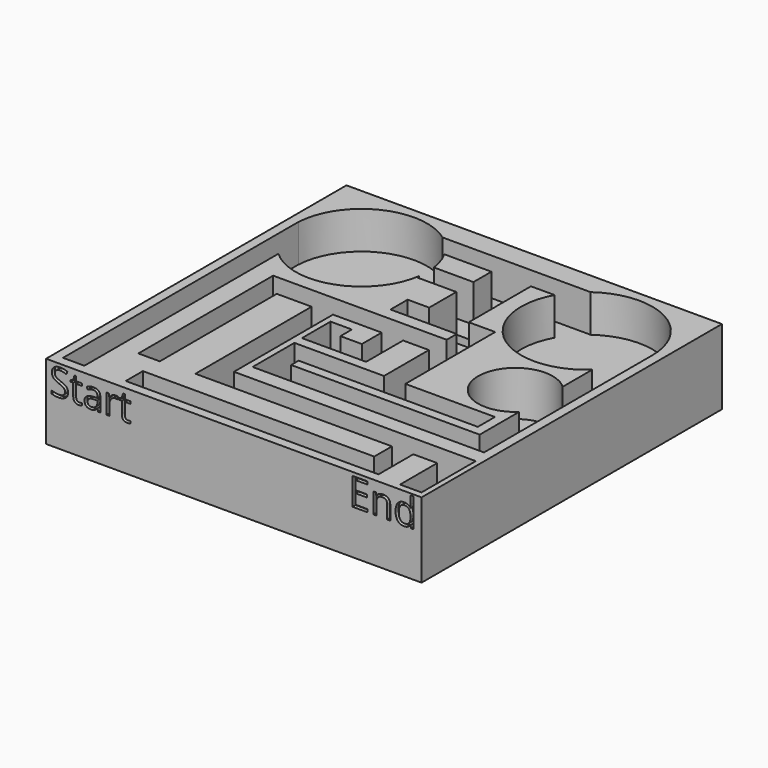
from build123d import *

# Parameters (mm, degrees)
F0_W           = 100
F0_H           = 100
F1_DEPTH       = 20
F2_W           = 10.5249598597
F2_H           = 5.9832503918
F2_W_2         = 17.6280021053
F2_H_2         = 5.7
F2_W_3         = 5.7
F2_H_3         = 38.9400205359
F2_H_4         = 28.7457114801
F2_H_5         = 3.8266098127
F2_H_6         = 12.3720951378
F2_W_4         = 38.370216731
F2_W_5         = 23.2461518608
F3_DEPTH       = 10
F4_R           = 9.9309063048
F4_W           = 10.5430610453
F4_H           = 9.0340993889
F5_DEPTH       = 12
F6_TEXT_SIZE   = 9.8178762772
F6_TEXT_SIZE_2 = 10.1638148971
F7_DEPTH       = 1
F8_TEXT_SIZE   = 18.6877515587
F9_DEPTH       = 1


# Not quite as in the source:
# - Text() gives the source's letters only with a copy of the font that has no kerning and outlines rounded to 1/6400 em; it was checked with that copy


with BuildPart() as f1:
    # F0 (on Top) → F1 (new body)
    with BuildSketch(Plane.XY):
        Rectangle(F0_W, F0_H)
    extrude(amount=-F1_DEPTH)

    # F2 (on face) → F3 (cut)
    with BuildSketch(Plane.XY):
        with BuildLine():
            ThreePointArc((-12.675344194, 27.528906881), (-12.5438910893, 28.7613468212), (-12.5, 30))
            ThreePointArc((-12.5, 30), (-12.5438910893, 31.2386531788), (-12.675344194, 32.471093119))
            Line((-12.675344194, 32.471093119), (-12.675344194, 27.528906881))
        make_face()
        with BuildLine():
            ThreePointArc((-12.675344194, 32.471093119), (-12.5438910893, 31.2386531788), (-12.5, 30))
            ThreePointArc((-12.5, 30), (-12.5438910893, 28.7613468212), (-12.675344194, 27.528906881))
            Line((-12.675344194, 27.528906881), (-12.675344194, 26.771093119))
            Line((-12.675344194, 26.771093119), (2.7480376884, 26.771093119))
            Line((2.7480376884, 26.771093119), (8.3745755255, 26.771093119))
            Line((8.3745755255, 26.771093119), (8.3745755255, 32.471093119))
            Line((8.3745755255, 32.471093119), (-2.1503843342, 32.471093119))
            Line((-2.1503843342, 32.471093119), (-12.675344194, 32.471093119))
        make_face()
        with BuildLine():
            Line((-12.675344194, 27.528906881), (-12.675344194, 32.471093119))
            ThreePointArc((-12.675344194, 32.471093119), (-13.4046274349, 35.553702317), (-14.67766089, 38.4543435108))
            Line((-14.67766089, 38.4543435108), (-19.7090058897, 38.4543435108))
            Line((-19.7090058897, 38.4543435108), (-19.7090058897, 44.1543435108))
            ThreePointArc((-19.7090058897, 44.1543435108), (-37.5622804937, 45.7816955279), (-47.4794772235, 30.8472756296))
            Line((-47.4794772235, 30.8472756296), (-41.8, 30.8472756296))
            Line((-41.8, 30.8472756296), (-41.8, 17.0767651109))
            ThreePointArc((-41.8, 17.0767651109), (-24.0888011081, 13.5285784566), (-12.675344194, 27.528906881))
        make_face()
        with BuildLine():
            Line((-19.7090058897, 38.4543435108), (-14.67766089, 38.4543435108))
            ThreePointArc((-14.67766089, 38.4543435108), (-16.8800453635, 41.5808803783), (-19.7090058897, 44.1543435108))
            Line((-19.7090058897, 44.1543435108), (-19.7090058897, 38.4543435108))
        make_face()
        with BuildLine():
            ThreePointArc((-19.7090058897, 44.1543435108), (-16.8800453635, 41.5808803783), (-14.67766089, 38.4543435108))
            Line((-14.67766089, 38.4543435108), (-2.1503843342, 38.4543435108))
            Line((-2.1503843342, 38.4543435108), (8.3745755255, 38.4543435108))
            Line((8.3745755255, 38.4543435108), (14.67766089, 38.4543435108))
            ThreePointArc((14.67766089, 38.4543435108), (16.8800453635, 41.5808803783), (19.7090058897, 44.1543435108))
            Line((19.7090058897, 44.1543435108), (-19.7090058897, 44.1543435108))
        make_face()
        with Locations((3.1120955956, 35.4627183149)):
            Rectangle(F2_W, F2_H)
        with BuildLine():
            Line((-41.8, 7.7384602059), (-41.8, 17.0767651109))
            ThreePointArc((-41.8, 17.0767651109), (-46.0117144819, 22.9377766002), (-47.5, 30.0000001007))
            Line((-47.5, 30.0000001007), (-47.5, -47.5))
            Line((-47.5, -47.5), (-41.8, -47.5))
            Line((-41.8, -47.5), (-41.8, 2.931000432))
            Line((-41.8, 2.931000432), (-41.8, 7.7384602059))
        make_face()
        with BuildLine():
            ThreePointArc((-47.5, 30.0000001007), (-46.0117144819, 22.9377766002), (-41.8, 17.0767651109))
            Line((-41.8, 17.0767651109), (-41.8, 30.8472756296))
            Line((-41.8, 30.8472756296), (-47.4794772235, 30.8472756296))
            ThreePointArc((-47.4794772235, 30.8472756296), (-47.4948685523, 30.423762123), (-47.5, 30.0000001007))
        make_face()
        with BuildLine():
            Line((-47.5, 30.8472756296), (-47.5, 30.0000001007))
            ThreePointArc((-47.5, 30.0000001007), (-47.4948685523, 30.423762123), (-47.4794772235, 30.8472756296))
            Line((-47.4794772235, 30.8472756296), (-47.5, 30.8472756296))
        make_face()
        with BuildLine():
            Line((19.8722742498, 44.1543435108), (19.7090058897, 44.1543435108))
            ThreePointArc((19.7090058897, 44.1543435108), (16.8800453635, 41.5808803783), (14.67766089, 38.4543435108))
            Line((14.67766089, 38.4543435108), (19.8722742498, 38.4543435108))
            Line((19.8722742498, 38.4543435108), (19.8722742498, 44.1543435108))
        make_face()
        with BuildLine():
            ThreePointArc((47.5, 30), (37.942216412, 45.5939474946), (19.7090058897, 44.1543435108))
            Line((19.7090058897, 44.1543435108), (19.8722742498, 44.1543435108))
            Line((19.8722742498, 44.1543435108), (19.8722742498, 38.4543435108))
            Line((19.8722742498, 38.4543435108), (14.67766089, 38.4543435108))
            ThreePointArc((14.67766089, 38.4543435108), (19.1649092176, 16.2577000565), (41.795897507, 17.0730203835))
            Line((41.795897507, 17.0730203835), (41.795897507, 29.621093119))
            Line((41.795897507, 29.621093119), (47.495897507, 29.621093119))
            ThreePointArc((47.495897507, 29.621093119), (47.4989743467, 29.8105354552), (47.5, 30))
        make_face()
        with BuildLine():
            Line((47.495897507, -0.2311933598), (47.495897507, 29.621093119))
            ThreePointArc((47.495897507, 29.621093119), (45.9331681134, 22.7623101841), (41.795897507, 17.0730203835))
            Line((41.795897507, 17.0730203835), (41.795897507, -0.2311933598))
            Line((41.795897507, -0.2311933598), (47.495897507, -0.2311933598))
        make_face()
        with BuildLine():
            ThreePointArc((41.795897507, 17.0730203835), (45.9331681134, 22.7623101841), (47.495897507, 29.621093119))
            Line((47.495897507, 29.621093119), (41.795897507, 29.621093119))
            Line((41.795897507, 29.621093119), (41.795897507, 17.0730203835))
        make_face()
        Polygon((47.495897507, -26.0778535157), (47.495897507, -0.2311933598), (41.795897507, -0.2311933598), (41.795897507, -20.3778535157), (41.795897507, -26.0778535157), align=None)
        Polygon((41.795897507, -26.0778535157), (41.795897507, -20.3778535157), (-8.432225886, -20.3778535157), (-14.132225886, -20.3778535157), (-14.132225886, -26.0778535157), align=None)
        Polygon((-14.132225886, -20.3778535157), (-8.432225886, -20.3778535157), (-8.432225886, -17.8778535157), (-8.432225886, -12.1778535157), (-14.132225886, -12.1778535157), align=None)
        Polygon((-8.432225886, -12.1778535157), (-8.432225886, -17.8778535157), (39.295897507, -17.8778535157), (39.295897507, -12.1778535157), (32.7667227619, -12.1778535157), (15.4318358105, -12.1778535157), (9.7318358105, -12.1778535157), align=None)
        Polygon((9.7318358105, 2.7795701072), (9.7318358105, -12.1778535157), (15.4318358105, -12.1778535157), (15.4318358105, 17.7369937301), (9.7318358105, 17.7369937301), (9.7318358105, 12.0369937301), (9.7318358105, 8.7082730606), align=None)
        Polygon((2.8549974695, 2.7795701072), (9.7318358105, 2.7795701072), (9.7318358105, 8.7082730606), (-36.4886954397, 8.7082730606), (-36.4886954397, 2.7795701072), (-30.7886954397, 2.7795701072), (-29.9770668119, 2.7795701072), (-26.0700903803, 2.7795701072), (-21.511951831, 2.7795701072), (-15.811951831, 2.7795701072), (-2.8450025305, 2.7795701072), align=None)
        Polygon((2.8549974695, -9.5266098127), (2.8549974695, 2.7795701072), (-2.8450025305, 2.7795701072), (-2.8450025305, -3.8266098127), (-2.8450025305, -9.5266098127), align=None)
        with Locations((0.9178347578, 14.8869937301)):
            Rectangle(F2_W_2, F2_H_2)
        with Locations((-33.6386954397, -16.6904401608)):
            Rectangle(F2_W_3, F2_H_3)
        with Locations((-18.661951831, -11.5932856329)):
            Rectangle(F2_W_3, F2_H_4)
        Polygon((-2.8450025305, -9.5266098127), (-2.8450025305, -3.8266098127), (-8.5450025305, -3.8266098127), (-14.2450025305, -3.8266098127), (-14.2450025305, -9.5266098127), align=None)
        Polygon((-15.811951831, -30.19637205), (-15.811951831, -25.9661413729), (-21.511951831, -25.9661413729), (-21.511951831, -35.89637205), (-15.811951831, -35.89637205), align=None)
        with Locations((-11.3950025305, -1.9133049063)):
            Rectangle(F2_W_3, F2_H_5)
        Polygon((48.5945235908, -30.19637205), (-15.811951831, -30.19637205), (-15.811951831, -35.89637205), (30.8276685918, -35.89637205), (36.5276685918, -35.89637205), (42.8945235908, -35.89637205), (48.5945235908, -35.89637205), align=None)
        Polygon((36.5276685918, -35.89637205), (30.8276685918, -35.89637205), (30.8276685918, -41.7903732538), (30.8276685918, -47.4903732538), (36.5276685918, -47.4903732538), align=None)
        with Locations((45.7445235908, -42.082419619)):
            Rectangle(F2_W_3, F2_H_6)
        with Locations((11.6425602263, -44.6403732538)):
            Rectangle(F2_W_4, F2_H_2)
        with Locations((-19.1656240696, -44.6403732538)):
            Rectangle(F2_W_5, F2_H_2)
    extrude(amount=-F3_DEPTH, mode=Mode.SUBTRACT)

    # F4 (on face) → F5 (cut)
    with BuildSketch(Plane.XY):
        with Locations((35.0043028593, 0)):
            Circle(F4_R)
        with Locations((3.1211461884, 22.2540434245)):
            Rectangle(F4_W, F4_H)
    extrude(amount=-F5_DEPTH, mode=Mode.SUBTRACT)

    # F6 (on face) → F7 (cut)
    with BuildSketch(Plane.XZ.offset(50)):
        with Locations((-49.0655650501, -7.9333089919)):
            Text('Start', F6_TEXT_SIZE, font='Open Sans', text_align=(TextAlign.LEFT, TextAlign.BOTTOM))
        with Locations((30.6139104166, -8.1823845654)):
            Text('End', F6_TEXT_SIZE_2, font='Open Sans', text_align=(TextAlign.LEFT, TextAlign.BOTTOM))
    extrude(amount=-F7_DEPTH, mode=Mode.SUBTRACT)

    # F8 (on face) → F9 (cut)
    with BuildSketch(Plane(origin=(0, 50, 0), x_dir=(-1, 0, 0), z_dir=(0, 1, 0))):
        with Locations((-25.4854211881, -17.0775916057)):
            Text('ACME', F8_TEXT_SIZE, font='Open Sans', text_align=(TextAlign.LEFT, TextAlign.BOTTOM))
    extrude(amount=-F9_DEPTH, mode=Mode.SUBTRACT)


solid = f1.part
